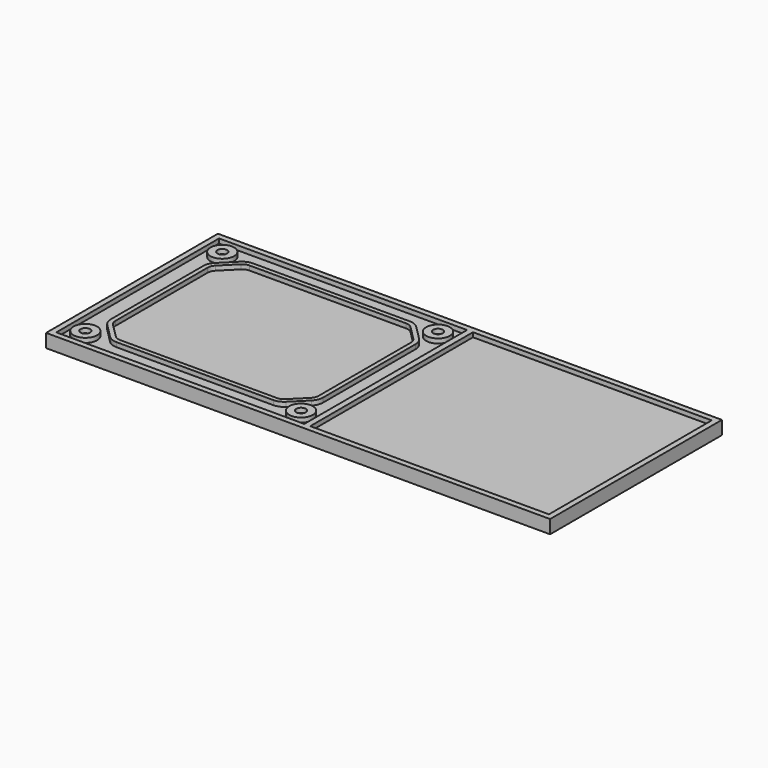
from build123d import *

# Parameters (mm, degrees)
F1_DEPTH = 2.25
F0_R     = 3.95
F0_R_2   = 1.6
F2_W     = 83.01
F2_H     = 68.1
F2_W_2   = 79.9
F3_DEPTH = 3


# Not quite as in the source:
# - a feature of the source that left no trace in its solid (it failed there, or was rolled back) is left out


with BuildPart() as f1:
    # F0 (on Top) → F1 (new body, symmetric)
    with BuildSketch(Plane.XY):
        Polygon((-84.35, -35.95), (84.35, -35.95), (84.35, 0), (82.45, 0), (82.45, -34.05), (2.55, -34.05), (2.55, 0), (0.56, 0), (0.56, -34.05), (-82.45, -34.05), (-82.45, 0), (-84.35, 0), align=None)
        Polygon((82.45, 0), (84.35, 0), (84.35, 35.95), (-84.35, 35.95), (-84.35, 0), (-82.45, 0), (-82.45, 34.05), (0.56, 34.05), (0.56, 0), (2.55, 0), (2.55, 34.05), (82.45, 34.05), align=None)
    extrude(amount=F1_DEPTH, both=True)

    # F2 (on face) → F3 (join)
    with BuildSketch(Plane(origin=(0, 0, -2.25), x_dir=(1, 0, 0), z_dir=(0, 0, -1))):
        with Locations((-40.945, 0)):
            Rectangle(F2_W, F2_H)
        with Locations((42.5, 0)):
            Rectangle(F2_W_2, F2_H)
    extrude(amount=-F3_DEPTH)


with BuildPart() as f1b:
    # F0 (on Top) → F1, piece 2 (new body, symmetric)
    with BuildSketch(Plane.XY):
        with Locations((-77.05, 28.65)):
            Circle(F0_R)
        with Locations((-77.05, 28.65)):
            Circle(F0_R_2, mode=Mode.SUBTRACT)
    extrude(amount=F1_DEPTH, both=True)


with BuildPart() as f1c:
    # F0 (on Top) → F1, piece 3 (new body, symmetric)
    with BuildSketch(Plane.XY):
        with Locations((-77.05, -28.65)):
            Circle(F0_R)
        with Locations((-77.05, -28.65)):
            Circle(F0_R_2, mode=Mode.SUBTRACT)
    extrude(amount=F1_DEPTH, both=True)


with BuildPart() as f1d:
    # F0 (on Top) → F1, piece 4 (new body, symmetric)
    with BuildSketch(Plane.XY):
        with Locations((-4.84, 28.65)):
            Circle(F0_R)
        with Locations((-4.84, 28.65)):
            Circle(F0_R_2, mode=Mode.SUBTRACT)
    extrude(amount=F1_DEPTH, both=True)


with BuildPart() as f1e:
    # F0 (on Top) → F1, piece 5 (new body, symmetric)
    with BuildSketch(Plane.XY):
        with Locations((-4.84, -28.65)):
            Circle(F0_R)
        with Locations((-4.84, -28.65)):
            Circle(F0_R_2, mode=Mode.SUBTRACT)
    extrude(amount=F1_DEPTH, both=True)


with BuildPart() as f1f:
    # F0 (on Top) → F1, piece 6 (new body, symmetric)
    with BuildSketch(Plane.XY):
        with BuildLine():
            Line((-75.95, 19.3073593129), (-75.95, 0))
            Line((-75.95, 0), (-74.45, 0))
            Line((-74.45, 0), (-74.45, 19.3073593129))
            ThreePointArc((-74.45, 19.3073593129), (-74.2216385975, 20.45540961), (-73.5713203436, 21.4286796564))
            Line((-73.5713203436, 21.4286796564), (-68.8286796564, 26.1713203436))
            ThreePointArc((-68.8286796564, 26.1713203436), (-67.85540961, 26.8216385975), (-66.7073593129, 27.05))
            Line((-66.7073593129, 27.05), (-14.1926406871, 27.05))
            ThreePointArc((-14.1926406871, 27.05), (-13.04459039, 26.8216385975), (-12.0713203436, 26.1713203436))
            Line((-12.0713203436, 26.1713203436), (-7.3286796564, 21.4286796564))
            ThreePointArc((-7.3286796564, 21.4286796564), (-6.6783614025, 20.45540961), (-6.45, 19.3073593129))
            Line((-6.45, 19.3073593129), (-6.45, 0))
            Line((-6.45, 0), (-4.95, 0))
            Line((-4.95, 0), (-4.95, 19.3073593129))
            ThreePointArc((-4.95, 19.3073593129), (-5.2925421037, 21.0294347585), (-6.2680194847, 22.4893398282))
            Line((-6.2680194847, 22.4893398282), (-11.0106601718, 27.2319805153))
            ThreePointArc((-11.0106601718, 27.2319805153), (-12.4705652415, 28.2074578963), (-14.1926406871, 28.55))
            Line((-14.1926406871, 28.55), (-66.7073593129, 28.55))
            ThreePointArc((-66.7073593129, 28.55), (-68.4294347585, 28.2074578963), (-69.8893398282, 27.2319805153))
            Line((-69.8893398282, 27.2319805153), (-74.6319805153, 22.4893398282))
            ThreePointArc((-74.6319805153, 22.4893398282), (-75.6074578963, 21.0294347585), (-75.95, 19.3073593129))
        make_face()
        with BuildLine():
            Line((-74.45, 0), (-75.95, 0))
            Line((-75.95, 0), (-75.95, -19.3073593129))
            ThreePointArc((-75.95, -19.3073593129), (-75.6074578963, -21.0294347585), (-74.6319805153, -22.4893398282))
            Line((-74.6319805153, -22.4893398282), (-69.8893398282, -27.2319805153))
            ThreePointArc((-69.8893398282, -27.2319805153), (-68.4294347585, -28.2074578963), (-66.7073593129, -28.55))
            Line((-66.7073593129, -28.55), (-14.1926406871, -28.55))
            ThreePointArc((-14.1926406871, -28.55), (-12.4705652415, -28.2074578963), (-11.0106601718, -27.2319805153))
            Line((-11.0106601718, -27.2319805153), (-6.2680194847, -22.4893398282))
            ThreePointArc((-6.2680194847, -22.4893398282), (-5.2925421037, -21.0294347585), (-4.95, -19.3073593129))
            Line((-4.95, -19.3073593129), (-4.95, 0))
            Line((-4.95, 0), (-6.45, 0))
            Line((-6.45, 0), (-6.45, -19.3073593129))
            ThreePointArc((-6.45, -19.3073593129), (-6.6783614025, -20.45540961), (-7.3286796564, -21.4286796564))
            Line((-7.3286796564, -21.4286796564), (-12.0713203436, -26.1713203436))
            ThreePointArc((-12.0713203436, -26.1713203436), (-13.04459039, -26.8216385975), (-14.1926406871, -27.05))
            Line((-14.1926406871, -27.05), (-66.7073593129, -27.05))
            ThreePointArc((-66.7073593129, -27.05), (-67.85540961, -26.8216385975), (-68.8286796564, -26.1713203436))
            Line((-68.8286796564, -26.1713203436), (-73.5713203436, -21.4286796564))
            ThreePointArc((-73.5713203436, -21.4286796564), (-74.2216385975, -20.45540961), (-74.45, -19.3073593129))
            Line((-74.45, -19.3073593129), (-74.45, 0))
        make_face()
    extrude(amount=F1_DEPTH, both=True)


solid = Compound([f1.part, f1b.part, f1c.part, f1d.part, f1e.part, f1f.part])
